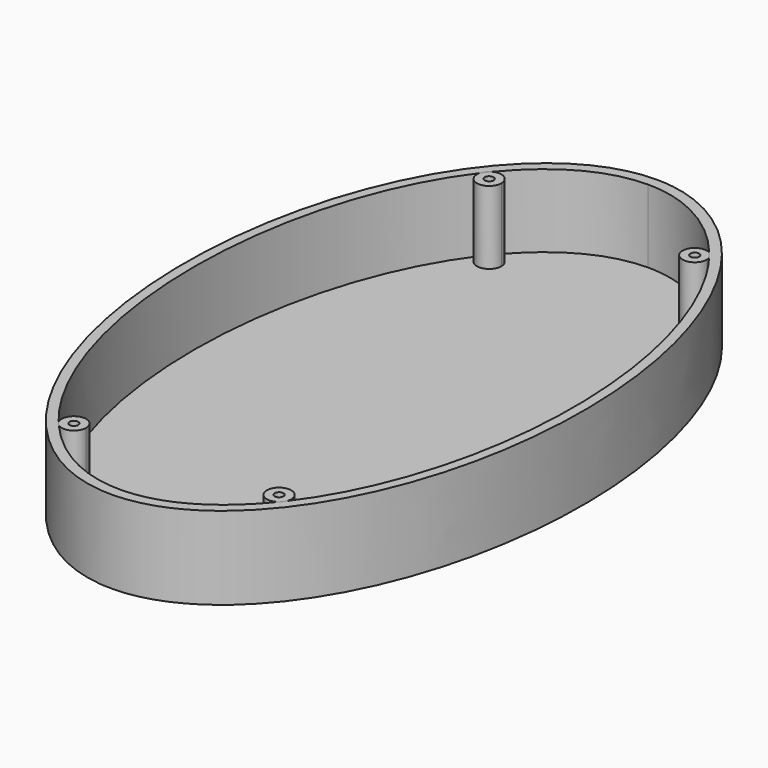
from build123d import *

# Parameters (mm, degrees)
F1_DEPTH  = 17
F3_DEPTH  = 15
F4_R      = 0.9
F5_DEPTH  = 15
F6_R      = 0.9
F7_DEPTH  = 15
F8_R      = 0.9
F9_DEPTH  = 15
F10_R     = 0.9
F11_DEPTH = 15
F13_R     = 0.9
F14_DEPTH = 9


with BuildPart() as f1:
    # F0 (on Top) → F1 (new body)
    with BuildSketch(Plane.XY):
        with BuildLine():
            add(Edge.make_bspline(
                [(-6.2171048485, 73.2565789297), (-77.2311879588, 73.2565789297), (-41.7241464036, -31.7434210703), (-6.2171048485, -136.7434210703), (29.2899367067, -31.7434210703), (64.7969782618, 73.2565789297), (-6.2171048485, 73.2565789297)],
                knots=[0, 0, 0, 2.0943951024, 2.0943951024, 4.1887902048, 4.1887902048, 6.2831853072, 6.2831853072, 6.2831853072], degree=2, weights=[1, 0.5, 1, 0.5, 1, 0.5, 1]))
        make_face()
    extrude(amount=F1_DEPTH)

    # F2 (on face) → F3 (cut)
    with BuildSketch(Plane.XY.offset(17)):
        with BuildLine():
            add(Edge.make_bspline(
                [(-6.2171048485, 71.0526332259), (-73.7670863437, 71.0526332259), (-39.9920955961, -30.6414482184), (-6.2171048485, -132.3355296627), (27.5578858991, -30.6414482184), (61.3328766467, 71.0526332259), (-6.2171048485, 71.0526332259)],
                knots=[0, 0, 0, 2.0943951024, 2.0943951024, 4.1887902048, 4.1887902048, 6.2831853072, 6.2831853072, 6.2831853072], degree=2, weights=[1, 0.5, 1, 0.5, 1, 0.5, 1]))
        make_face()
    extrude(amount=-F3_DEPTH, mode=Mode.SUBTRACT)

    # F4 (on face) → F5 (join)
    with BuildSketch(Plane.XY.offset(2)):
        with BuildLine():
            ThreePointArc((-29.7756858862, 57.2855702673), (-27.6492449133, 54.2060390081), (-24.8481921157, 56.6878462554))
            ThreePointArc((-24.8481921157, 56.6878462554), (-26.0432758657, 58.8202612198), (-28.48594698, 58.9139446065))
            add(Edge.make_bspline(
                [(-28.48594698, 58.9139446065), (-29.1403899926, 58.1226714215), (-29.7756858862, 57.2855702673)],
                knots=[0.6420928407, 0.6420928407, 0.6420928407, 0.6808401148, 0.6808401148, 0.6808401148], degree=2, weights=[0.7874125542, 0.783834135, 0.7805979828]))
        make_face()
        with Locations((-27.3481921157, 56.6878462554)):
            Circle(F4_R, mode=Mode.SUBTRACT)
        with BuildLine():
            add(Edge.make_bspline(
                [(-28.48594698, 58.9139446065), (-29.1403899926, 58.1226714215), (-29.7756858862, 57.2855702673)],
                knots=[0.6420928407, 0.6420928407, 0.6420928407, 0.6808401148, 0.6808401148, 0.6808401148], degree=2, weights=[0.7874125542, 0.783834135, 0.7805979828]))
            ThreePointArc((-28.48594698, 58.9139446065), (-29.3079498058, 58.2400542943), (-29.7756858862, 57.2855702673))
        make_face()
    extrude(amount=F5_DEPTH)

    # F6 (on face) → F7 (join)
    with BuildSketch(Plane.XY.offset(2)):
        with BuildLine():
            ThreePointArc((16.1916939477, 58.7439345546), (12.7793422864, 55.3266057789), (17.4437982507, 56.577657488))
            ThreePointArc((17.4437982507, 56.577657488), (17.4180855063, 56.9352921855), (17.3414761892, 57.2855702673))
            add(Edge.make_bspline(
                [(17.3414761892, 57.2855702673), (16.7742405528, 58.0329914466), (16.1916939477, 58.7439345546)],
                knots=[5.6023451924, 5.6023451924, 5.6023451924, 5.6369260508, 5.6369260508, 5.6369260508], degree=2, weights=[0.7805979828, 0.7834861581, 0.7866469513]))
        make_face()
        with Locations((14.9437982507, 56.577657488)):
            Circle(F6_R, mode=Mode.SUBTRACT)
    extrude(amount=F7_DEPTH)

    # F8 (on face) → F9 (join)
    with BuildSketch(Plane.XY.offset(2)):
        with BuildLine():
            ThreePointArc((-27.8172974331, -53.191482885), (-25.1847662143, -53.4621797963), (-23.7840667271, -51.2168427654))
            ThreePointArc((-23.7840667271, -51.2168427654), (-26.8945171213, -48.792518052), (-28.48594698, -52.4007867471))
            add(Edge.make_bspline(
                [(-28.48594698, -52.4007867471), (-28.1539802485, -52.8021606908), (-27.8172974331, -53.191482885)],
                knots=[2.5728398269, 2.5728398269, 2.5728398269, 2.5934282254, 2.5934282254, 2.5934282254], degree=2, weights=[0.8237445465, 0.8210750527, 0.8185021925]))
        make_face()
        with Locations((-26.2840667271, -51.2168427654)):
            Circle(F8_R, mode=Mode.SUBTRACT)
    extrude(amount=F9_DEPTH)

    # F10 (on face) → F11 (join)
    with BuildSketch(Plane.XY.offset(2)):
        with BuildLine():
            ThreePointArc((17.2071260982, -50.948647347), (17.3423414514, -50.4905518475), (17.3879683871, -50.0151016807))
            ThreePointArc((17.3879683871, -50.0151016807), (12.6660564501, -48.8691927208), (16.3374825114, -52.0519887181))
            add(Edge.make_bspline(
                [(16.3374825114, -52.0519887181), (16.7766850943, -51.5107523345), (17.2071260982, -50.948647347)],
                knots=[3.7192756497, 3.7192756497, 3.7192756497, 3.746975358, 3.746975358, 3.746975358], degree=2, weights=[0.8260785, 0.8297264389, 0.8335492953]))
        make_face()
        with Locations((14.8879683871, -50.0151016807)):
            Circle(F10_R, mode=Mode.SUBTRACT)
        with BuildLine():
            add(Edge.make_bspline(
                [(16.3374825114, -52.0519887181), (16.7766850943, -51.5107523345), (17.2071260982, -50.948647347)],
                knots=[3.7192756497, 3.7192756497, 3.7192756497, 3.746975358, 3.746975358, 3.746975358], degree=2, weights=[0.8260785, 0.8297264389, 0.8335492953]))
            ThreePointArc((16.3374825114, -52.0519887181), (16.8513996683, -51.5626602753), (17.2071260982, -50.948647347))
        make_face()
    extrude(amount=F11_DEPTH)

    # F13 (on face) → F14 (cut)
    with BuildSketch(Plane.XY.offset(17)):
        with Locations((-27.3481921157, 56.6878462554)):
            Circle(F13_R)
        with Locations((14.9437982507, 56.577657488)):
            Circle(F13_R)
        with Locations((-26.2840667271, -51.2168427654)):
            Circle(F13_R)
        with Locations((14.8879683871, -50.0151016807)):
            Circle(F13_R)
    extrude(amount=-F14_DEPTH, mode=Mode.SUBTRACT)


solid = f1.part
